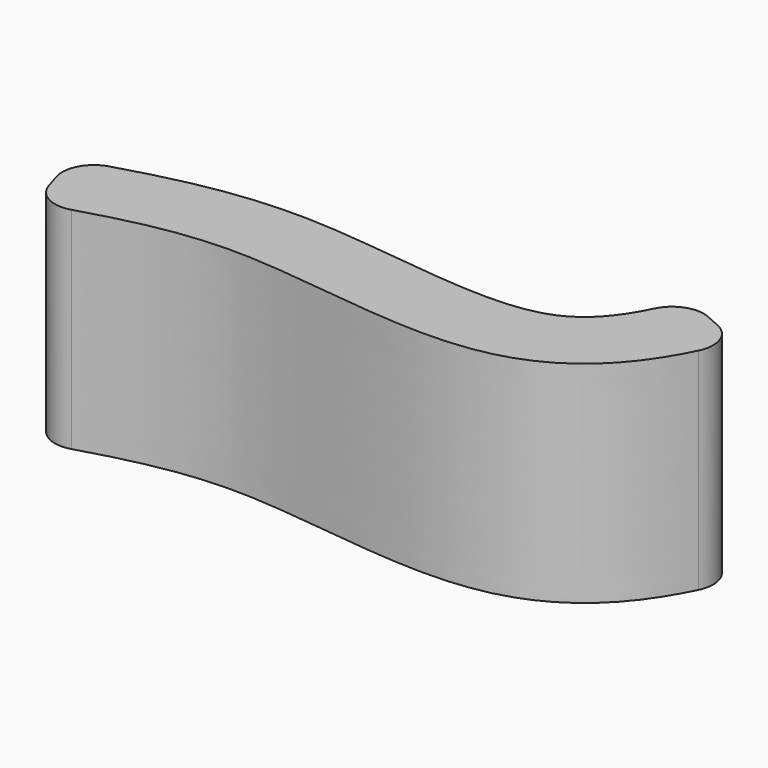
from build123d import *

# Parameters (mm, degrees)
F1_DEPTH = 50.8
F2_R     = 7.62


# Not quite as in the source:
# - the dataset's text gives a spline's control points without its knots; the knots are read off the source's solid


with BuildPart() as f1:
    # F0 (on Top) → F1 (new body)
    with BuildSketch(Plane.XY):
        with BuildLine():
            add(Edge.make_bspline(
                [(-60.944698751, 25.0633750111), (-45.7793490355, 29.7747773681), (-13.9600111377, 39.6600557418), (52.5503573555, 22.5129103077), (62.0745263261, 44.2466254476), (65.8716857433, 52.911568433)],
                knots=[0, 0, 0, 0, 0.3538232256, 0.7423779196, 1, 1, 1, 1], degree=3))
            Line((-60.944698751, 25.0633750111), (-55.2929164482, 6.8710728807))
            add(Edge.make_bspline(
                [(-55.2929164482, 6.8710728807), (-52.6140805534, 7.7033038537), (-47.4018926145, 9.3216145558), (-39.8812064113, 11.4599835905), (-33.7309143498, 12.9050992109), (-28.786328872, 13.8133593735), (-25.0381264341, 14.3598557381), (-21.2209235546, 14.7600271905), (-17.9562000554, 14.9607026798), (-15.2780901655, 15.0339227144), (-13.5728145637, 15.0414720085), (-12.1886095674, 15.0234734602), (-10.7871900479, 14.9888942675), (-8.9608161671, 14.9139701297), (-6.6734196362, 14.777094689), (-3.5073038309, 14.5377383447), (0.6395111781, 14.1444456971), (5.8438148043, 13.5682562387), (11.2137603043, 12.9395763815), (16.6986316777, 12.3136570181), (22.2601288935, 11.7494341891), (27.874607408, 11.3110698362), (33.5371111559, 11.0724127396), (38.3117706057, 11.1160284257), (42.1895309058, 11.3615597133), (45.1357695567, 11.6738573232), (48.129006294, 12.141988219), (50.6694852802, 12.6913928111), (52.7311013888, 13.2486701903), (54.0315996583, 13.6515527053), (55.0779843338, 14.009843186), (55.8669552145, 14.298012218), (56.6538003886, 14.6043360697), (58.2057168856, 15.2466006567), (60.4616240485, 16.3243567042), (63.2791892362, 17.9768086998), (65.881457239, 19.8076647102), (69.0445974475, 22.4299995717), (72.4118941025, 25.9363734821), (75.608842099, 30.2136170314), (78.1408898176, 34.3749839674), (80.1842586198, 38.3192081065), (81.8837517412, 41.9864350032), (82.8592586587, 44.2143404913), (83.3198606056, 45.26541293)],
                knots=[0, 0, 0, 0, 0.0625, 0.125, 0.1875, 0.21875, 0.25, 0.28125, 0.3125, 0.328125, 0.34375, 0.3515625, 0.359375, 0.375, 0.390625, 0.40625, 0.4375, 0.46875, 0.5, 0.53125, 0.5625, 0.59375, 0.625, 0.65625, 0.671875, 0.6875, 0.703125, 0.71875, 0.7265625, 0.734375, 0.73828125, 0.7421875, 0.74609375, 0.75, 0.765625, 0.78125, 0.796875, 0.8125, 0.84375, 0.875, 0.90625, 0.9375, 0.96875, 1, 1, 1, 1], degree=3))
            Line((83.3198606056, 45.26541293), (65.8716857433, 52.911568433))
        make_face()
    extrude(amount=F1_DEPTH)

    # F2
    f2_edges = [f1.edges().sort_by_distance(p)[0] for p in [
        (65.871686, 52.911568, 25.4),
        (83.319861, 45.265413, 25.4),
        (-60.944699, 25.063375, 25.4),
        (-55.292916, 6.871073, 25.4),
    ]]
    fillet(f2_edges, radius=F2_R)


solid = f1.part
